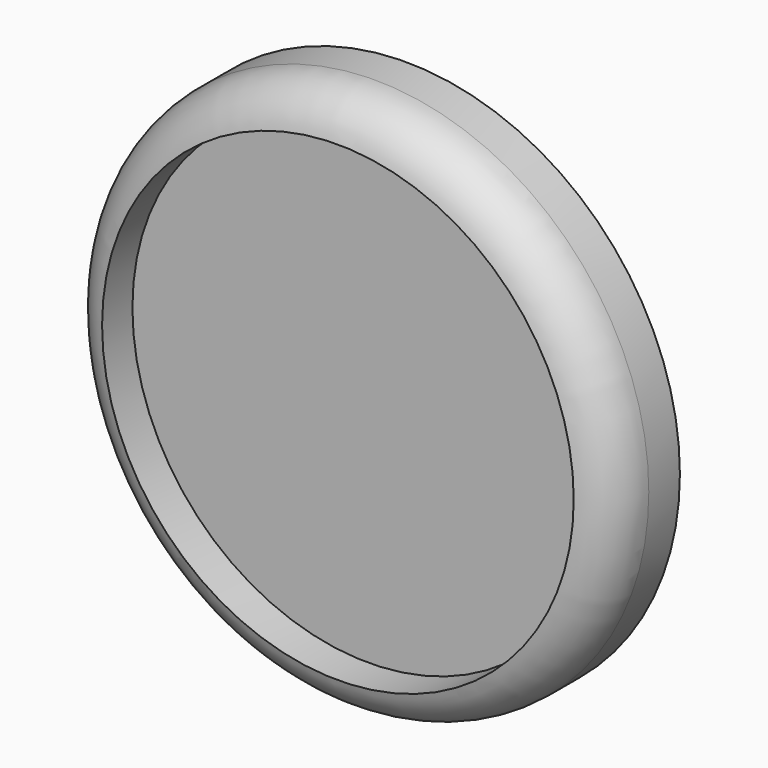
from build123d import *

# Parameters (mm, degrees)
F0_R     = 24.875
F1_DEPTH = 5
F0_R_2   = 28.875
F2_DEPTH = 9


# Not quite as in the source:
# - a fillet or chamfer that OpenCascade refuses, or shapes differently, is made with other operations: its cross-section is extruded or revolved along the edge and cut away or added


with BuildPart() as f1:
    # F0 (on Front) → F1 (new body)
    with BuildSketch(Plane.XZ):
        Circle(F0_R)
    extrude(amount=F1_DEPTH)


with BuildPart() as f2:
    # F0 (on Front) → F2 (new body)
    with BuildSketch(Plane.XZ):
        Circle(F0_R_2)
        Circle(F0_R, mode=Mode.SUBTRACT)
    extrude(amount=F2_DEPTH)

    # F3: fillet of radius 5 on 1 edges, made by hand

    # F3_s1 → F3_t2 (revolve, cut)
    with BuildSketch(Plane.XY):
        with BuildLine():
            ThreePointArc((28.875, -4.1010205144), (27.7479833462, -7.2632981746), (24.875, -9))
            Line((24.875, -9), (28.875, -9))
            Line((28.875, -9), (28.875, -4.1010205144))
        make_face()
    revolve(axis=Axis((0, -9, 0), (0, -1, 0)), mode=Mode.SUBTRACT)


solid = Compound([f1.part, f2.part])
